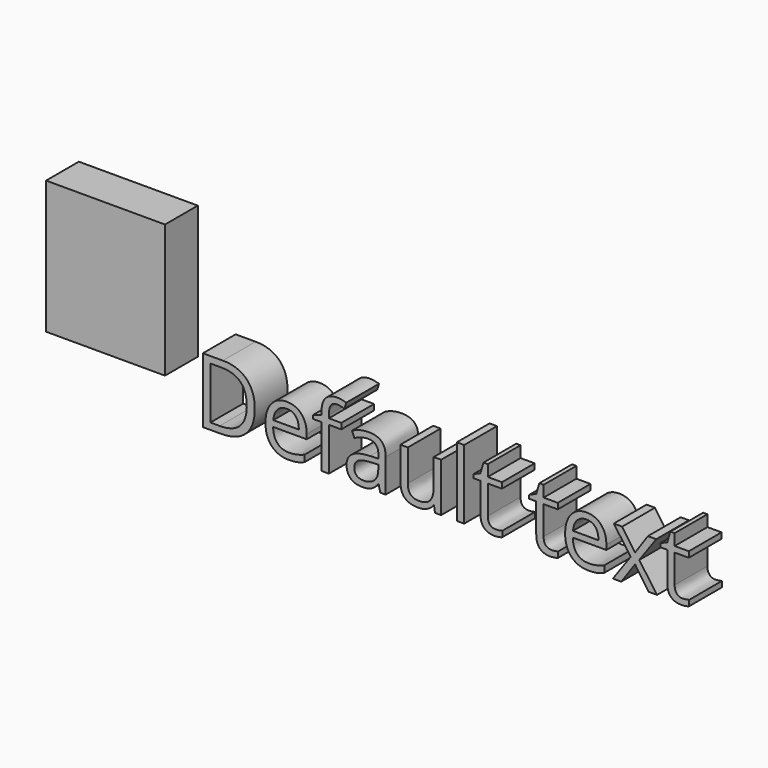
from build123d import *

# Parameters (mm, degrees)
F0_W         = 72.597656399
F0_H         = 81.2165215611
F1_DEPTH     = 25
F2_TEXT_SIZE = 55.6197741793
F3_DEPTH     = 25


# Not quite as in the source:
# - Text() gives the source's letters only with a copy of the font that has no kerning and outlines rounded to 1/6400 em; it was checked with that copy


with BuildPart() as f1:
    # F0 (on Front) → F1 (new body)
    with BuildSketch(Plane.XZ):
        with Locations((-11.2793128937, 40.6082607806)):
            Rectangle(F0_W, F0_H)
    extrude(amount=F1_DEPTH)


with BuildPart() as f3:
    # F2 (on Front) → F3 (new body)
    with BuildSketch(Plane.XZ):
        with Locations((42.656224221, -20.1445743442)):
            Text('Default text', F2_TEXT_SIZE, font='Open Sans', text_align=(TextAlign.LEFT, TextAlign.BOTTOM))
    extrude(amount=F3_DEPTH)


solid = Compound([f1.part, f3.part])
